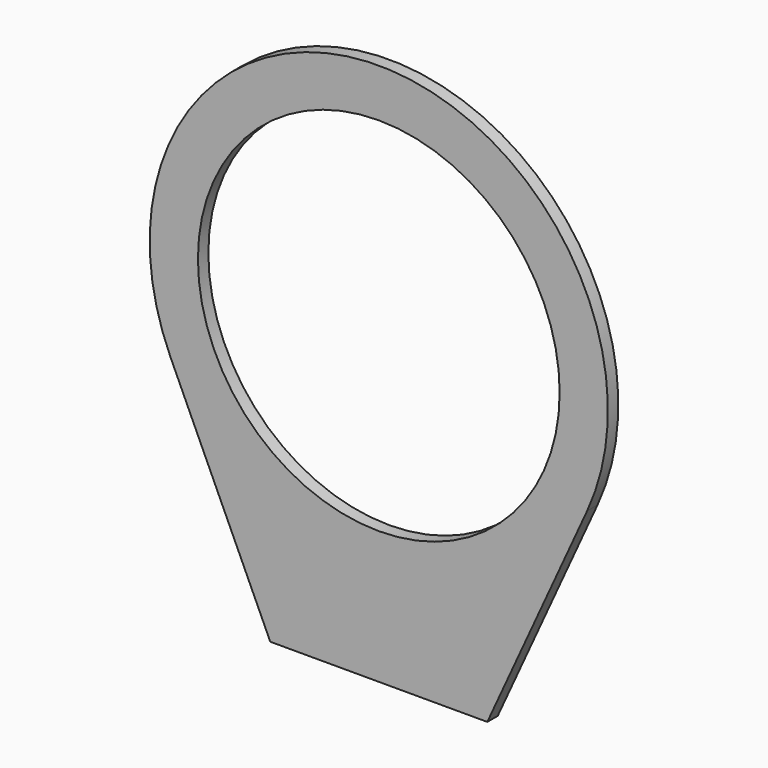
from build123d import *

# Parameters (mm, degrees)
F0_R     = 47.625
F1_DEPTH = 3.429


# Not quite as in the source:
# - ends of sketch curves that miss each other by under 0.0002 mm in the source are joined


with BuildPart() as f1:
    # F0 (on Front) → F1 (new body)
    with BuildSketch(Plane.XZ):
        with BuildLine():
            Line((-235.938695, 504.0320628), (-209.655918, 446.5764754))
            Line((-209.655918, 446.5764754), (-152.505918, 446.5764754))
            Line((-152.505918, 446.5764754), (-126.223141, 504.0320628))
            ThreePointArc((-126.223141, 504.0320628), (-181.080918, 589.4514754), (-235.938695, 504.0320628))
        make_face()
        with Locations((-181.080918, 529.1264754)):
            Circle(F0_R, mode=Mode.SUBTRACT)
    extrude(amount=F1_DEPTH)


solid = f1.part
